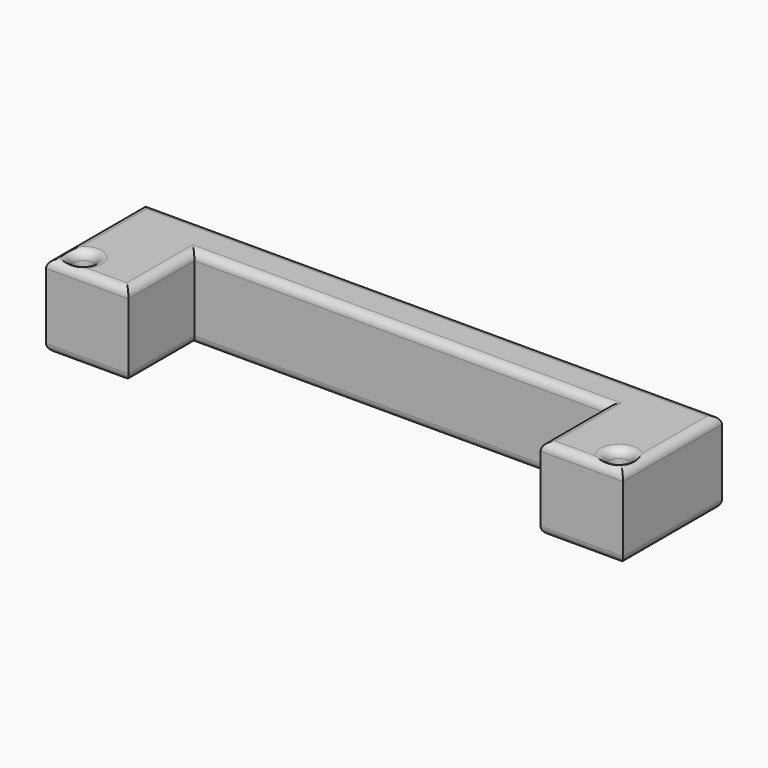
from build123d import *

# Parameters (mm, degrees)
F1_DEPTH     = 20
F3_D         = 5
F5_T1_DEPTH  = 150
F5_T3_DEPTH  = 40
F5_T5_DEPTH  = 30
F5_T7_DEPTH  = 25
F5_T9_DEPTH  = 100
F5_T11_DEPTH = 30
F5_T25_DEPTH = 105
F5_T29_DEPTH = 30
F5_T36_DEPTH = 30
F5_T40_DEPTH = 105
F5_T47_DEPTH = 30
F5_T51_DEPTH = 105
F5_T58_DEPTH = 105
F5_T62_DEPTH = 30


# Not quite as in the source:
# - a fillet or chamfer that OpenCascade refuses, or shapes differently, is made with other operations: its cross-section is extruded or revolved along the edge and cut away or added


with BuildPart() as f1:
    # F0 (on Top) → F1 (new body)
    with BuildSketch(Plane.XY):
        Polygon((70, 30), (0, 30), (0, 20), (50, 20), (50, 0), (70, 0), align=None)
    extrude(amount=F1_DEPTH)

    # F3 (through all)
    with Locations(Plane(origin=(0, 0, 0), x_dir=(1, 0, 0), z_dir=(0, 0, -1))):
        with Locations((65, -5)):
            Hole(F3_D / 2)

    # F4: F1 across face


with BuildPart() as f1_1:
    add(f1.part)
    add(f1.part.mirror(Plane(origin=(0, 25, 10), x_dir=(0, -1, 0), z_dir=(-1, 0, 0))))

    # F5: fillet of radius 2 on 20 edges, made by hand

    # F5_s2 → F5_t1 (cut)
    with BuildSketch(Plane.YZ.offset(-75)):
        with BuildLine():
            ThreePointArc((30, 18), (29.4142135624, 19.4142135624), (28, 20))
            Line((28, 20), (30, 20))
            Line((30, 20), (30, 18))
        make_face()
        with BuildLine():
            ThreePointArc((30, 2), (29.4142135624, 0.5857864376), (28, 0))
            Line((28, 0), (30, 0))
            Line((30, 0), (30, 2))
        make_face()
    extrude(amount=F5_T1_DEPTH, mode=Mode.SUBTRACT)

    # F5_s4 → F5_t3 (cut)
    with BuildSketch(Plane.XZ.offset(-35)):
        with BuildLine():
            ThreePointArc((-70, 18), (-69.4142135624, 19.4142135624), (-68, 20))
            Line((-68, 20), (-70, 20))
            Line((-70, 20), (-70, 18))
        make_face()
        with BuildLine():
            ThreePointArc((68, 20), (69.4142135624, 19.4142135624), (70, 18))
            Line((70, 18), (70, 20))
            Line((70, 20), (68, 20))
        make_face()
        with BuildLine():
            ThreePointArc((-68, 0), (-69.4142135624, 0.5857864376), (-70, 2))
            Line((-70, 2), (-70, 0))
            Line((-70, 0), (-68, 0))
        make_face()
        with BuildLine():
            ThreePointArc((68, 0), (69.4142135624, 0.5857864376), (70, 2))
            Line((70, 2), (70, 0))
            Line((70, 0), (68, 0))
        make_face()
    extrude(amount=F5_T3_DEPTH, mode=Mode.SUBTRACT)

    # F5_s6 → F5_t5 (cut)
    with BuildSketch(Plane.YZ.offset(-75)):
        with BuildLine():
            ThreePointArc((0, 18), (0.5857864376, 19.4142135624), (2, 20))
            Line((2, 20), (0, 20))
            Line((0, 20), (0, 18))
        make_face()
        with BuildLine():
            ThreePointArc((2, 0), (0.5857864376, 0.5857864376), (0, 2))
            Line((0, 2), (0, 0))
            Line((0, 0), (2, 0))
        make_face()
    extrude(amount=F5_T5_DEPTH, mode=Mode.SUBTRACT)

    # F5_s8 → F5_t7 (cut)
    with BuildSketch(Plane.XZ.offset(-20)):
        with BuildLine():
            ThreePointArc((-50, 18), (-50.5857864376, 19.4142135624), (-52, 20))
            Line((-52, 20), (-50, 20))
            Line((-50, 20), (-50, 18))
        make_face()
        with BuildLine():
            ThreePointArc((50, 18), (50.5857864376, 19.4142135624), (52, 20))
            Line((52, 20), (50, 20))
            Line((50, 20), (50, 18))
        make_face()
        with BuildLine():
            ThreePointArc((-52, 0), (-50.5857864376, 0.5857864376), (-50, 2))
            Line((-50, 2), (-50, 0))
            Line((-50, 0), (-52, 0))
        make_face()
        with BuildLine():
            ThreePointArc((52, 0), (50.5857864376, 0.5857864376), (50, 2))
            Line((50, 2), (50, 0))
            Line((50, 0), (52, 0))
        make_face()
    extrude(amount=F5_T7_DEPTH, mode=Mode.SUBTRACT)

    # F5_s10 → F5_t9 (cut)
    with BuildSketch(Plane.YZ.offset(-50)):
        with BuildLine():
            ThreePointArc((20, 18), (20.5857864376, 19.4142135624), (22, 20))
            Line((22, 20), (20, 20))
            Line((20, 20), (20, 18))
        make_face()
        with BuildLine():
            ThreePointArc((22, 0), (20.5857864376, 0.5857864376), (20, 2))
            Line((20, 2), (20, 0))
            Line((20, 0), (22, 0))
        make_face()
    extrude(amount=F5_T9_DEPTH, mode=Mode.SUBTRACT)

    # F5_s12 → F5_t11 (cut)
    with BuildSketch(Plane.YZ.offset(45)):
        with BuildLine():
            ThreePointArc((0, 18), (0.5857864376, 19.4142135624), (2, 20))
            Line((2, 20), (0, 20))
            Line((0, 20), (0, 18))
        make_face()
        with BuildLine():
            ThreePointArc((2, 0), (0.5857864376, 0.5857864376), (0, 2))
            Line((0, 2), (0, 0))
            Line((0, 0), (2, 0))
        make_face()
    extrude(amount=F5_T11_DEPTH, mode=Mode.SUBTRACT)

    # F5_s13 → F5_t14 (revolve, cut)
    with BuildSketch(Plane.XZ.offset(-5)):
        with BuildLine():
            ThreePointArc((67.5, 18), (68.0857864376, 19.4142135624), (69.5, 20))
            Line((69.5, 20), (67.5, 20))
            Line((67.5, 20), (67.5, 18))
        make_face()
    revolve(axis=Axis((65, 5, 20), (0, 0, -1)), mode=Mode.SUBTRACT)

    # F5_s15 → F5_t16 (revolve, cut)
    with BuildSketch(Plane.XZ.offset(-5)):
        with BuildLine():
            ThreePointArc((-67.5, 18), (-68.0857864376, 19.4142135624), (-69.5, 20))
            Line((-69.5, 20), (-67.5, 20))
            Line((-67.5, 20), (-67.5, 18))
        make_face()
    revolve(axis=Axis((-65, 5, 20), (0, 0, 1)), mode=Mode.SUBTRACT)

    # F5_s17 → F5_t18 (revolve, cut)
    with BuildSketch(Plane.XZ.offset(-5)):
        with BuildLine():
            ThreePointArc((69.5, 0), (68.0857864376, 0.5857864376), (67.5, 2))
            Line((67.5, 2), (67.5, 0))
            Line((67.5, 0), (69.5, 0))
        make_face()
    revolve(axis=Axis((65, 5, 0), (0, 0, -1)), mode=Mode.SUBTRACT)

    # F5_s19 → F5_t20 (revolve, cut)
    with BuildSketch(Plane.XZ.offset(-5)):
        with BuildLine():
            ThreePointArc((-69.5, 0), (-68.0857864376, 0.5857864376), (-67.5, 2))
            Line((-67.5, 2), (-67.5, 0))
            Line((-67.5, 0), (-69.5, 0))
        make_face()
    revolve(axis=Axis((-65, 5, 0), (0, 0, 1)), mode=Mode.SUBTRACT)


with BuildPart() as f5_tool23:
    # F5_s24 → F5_t25 (new body)
    with BuildSketch(Plane.YZ.offset(-55)):
        with BuildLine():
            ThreePointArc((20, 18), (20.5857864376, 19.4142135624), (22, 20))
            Line((22, 20), (20, 20))
            Line((20, 20), (20, 18))
        make_face()
    extrude(amount=F5_T25_DEPTH)

    split(bisect_by=Plane.YZ.offset(-50), keep=Keep.BOTTOM)


with BuildPart() as f5_tool27:
    # F5_s28 → F5_t29 (new body)
    with BuildSketch(Plane.XZ.offset(-25)):
        with BuildLine():
            ThreePointArc((-50, 18), (-50.5857864376, 19.4142135624), (-52, 20))
            Line((-52, 20), (-50, 20))
            Line((-50, 20), (-50, 18))
        make_face()
    extrude(amount=F5_T29_DEPTH)

    split(bisect_by=Plane.XZ.offset(-20), keep=Keep.BOTTOM)


with BuildPart() as f5_tool23_1:
    add(f5_tool23.part)

    # F5_t31: intersect F5_tool27
    add(f5_tool27.part, mode=Mode.INTERSECT)


with BuildPart() as f1_2:
    add(f1_1.part)

    # F5_t21: cut F5_tool23
    add(f5_tool23_1.part, mode=Mode.SUBTRACT)


with BuildPart() as f5_tool34:
    # F5_s35 → F5_t36 (new body)
    with BuildSketch(Plane.XZ.offset(-25)):
        with BuildLine():
            ThreePointArc((50, 18), (50.5857864376, 19.4142135624), (52, 20))
            Line((52, 20), (50, 20))
            Line((50, 20), (50, 18))
        make_face()
    extrude(amount=F5_T36_DEPTH)

    split(bisect_by=Plane.XZ.offset(-20), keep=Keep.BOTTOM)


with BuildPart() as f5_tool38:
    # F5_s39 → F5_t40 (new body)
    with BuildSketch(Plane.YZ.offset(-50)):
        with BuildLine():
            ThreePointArc((20, 18), (20.5857864376, 19.4142135624), (22, 20))
            Line((22, 20), (20, 20))
            Line((20, 20), (20, 18))
        make_face()
    extrude(amount=F5_T40_DEPTH)

    split(bisect_by=Plane.YZ.offset(50), keep=Keep.TOP)


with BuildPart() as f5_tool34_1:
    add(f5_tool34.part)

    # F5_t42: intersect F5_tool38
    add(f5_tool38.part, mode=Mode.INTERSECT)


with BuildPart() as f1_3:
    add(f1_2.part)

    # F5_t32: cut F5_tool34
    add(f5_tool34_1.part, mode=Mode.SUBTRACT)


with BuildPart() as f5_tool45:
    # F5_s46 → F5_t47 (new body)
    with BuildSketch(Plane.XZ.offset(-25)):
        with BuildLine():
            ThreePointArc((-52, 0), (-50.5857864376, 0.5857864376), (-50, 2))
            Line((-50, 2), (-50, 0))
            Line((-50, 0), (-52, 0))
        make_face()
    extrude(amount=F5_T47_DEPTH)

    split(bisect_by=Plane.XZ.offset(-20), keep=Keep.BOTTOM)


with BuildPart() as f5_tool49:
    # F5_s50 → F5_t51 (new body)
    with BuildSketch(Plane.YZ.offset(50)):
        with BuildLine():
            ThreePointArc((22, 0), (20.5857864376, 0.5857864376), (20, 2))
            Line((20, 2), (20, 0))
            Line((20, 0), (22, 0))
        make_face()
    extrude(amount=-F5_T51_DEPTH)

    split(bisect_by=Plane.YZ.offset(-50), keep=Keep.BOTTOM)


with BuildPart() as f5_tool45_1:
    add(f5_tool45.part)

    # F5_t53: intersect F5_tool49
    add(f5_tool49.part, mode=Mode.INTERSECT)


with BuildPart() as f1_4:
    add(f1_3.part)

    # F5_t43: cut F5_tool45
    add(f5_tool45_1.part, mode=Mode.SUBTRACT)


with BuildPart() as f5_tool56:
    # F5_s57 → F5_t58 (new body)
    with BuildSketch(Plane.YZ.offset(55)):
        with BuildLine():
            ThreePointArc((22, 0), (20.5857864376, 0.5857864376), (20, 2))
            Line((20, 2), (20, 0))
            Line((20, 0), (22, 0))
        make_face()
    extrude(amount=-F5_T58_DEPTH)

    split(bisect_by=Plane.YZ.offset(50), keep=Keep.TOP)


with BuildPart() as f5_tool60:
    # F5_s61 → F5_t62 (new body)
    with BuildSketch(Plane.XZ.offset(-25)):
        with BuildLine():
            ThreePointArc((52, 0), (50.5857864376, 0.5857864376), (50, 2))
            Line((50, 2), (50, 0))
            Line((50, 0), (52, 0))
        make_face()
    extrude(amount=F5_T62_DEPTH)

    split(bisect_by=Plane.XZ.offset(-20), keep=Keep.BOTTOM)


with BuildPart() as f5_tool56_1:
    add(f5_tool56.part)

    # F5_t64: intersect F5_tool60
    add(f5_tool60.part, mode=Mode.INTERSECT)


with BuildPart() as f1_5:
    add(f1_4.part)

    # F5_t54: cut F5_tool56
    add(f5_tool56_1.part, mode=Mode.SUBTRACT)


solid = f1_5.part
